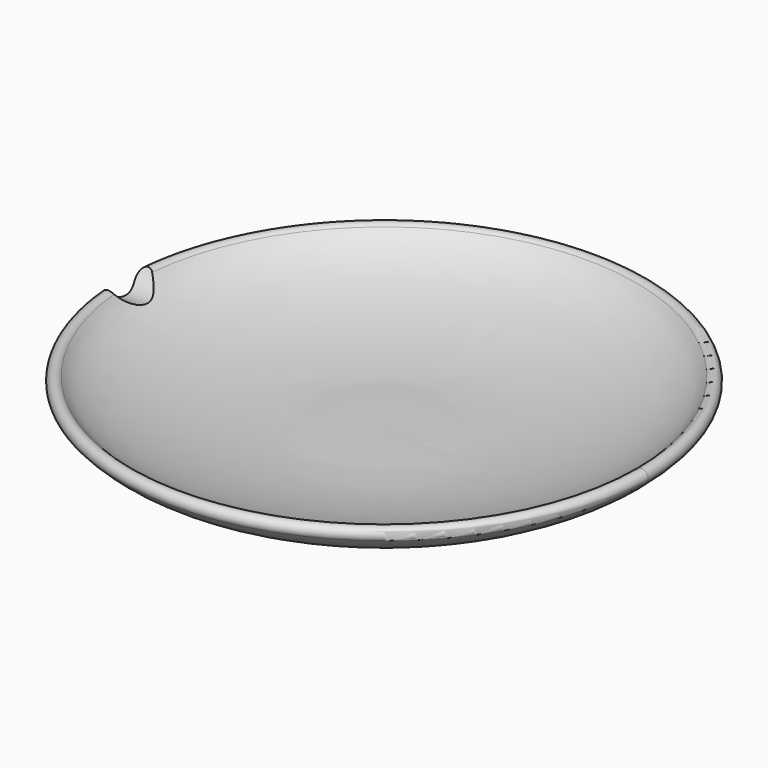
from build123d import *

# Parameters (mm, degrees)
F2_R     = 90.375022763
F3_DEPTH = 2.54
F4_R     = 6.7588472291
F5_DEPTH = 68.326


# Not quite as in the source:
# - the dataset's text gives a spline's control points without its knots; the knots are read off the source's solid


with BuildPart() as f1:
    # F0 (on Front) → F1 (revolve)
    with BuildSketch(Plane.XZ):
        with BuildLine():
            Line((0, 3.175), (0, 0))
            add(Edge.make_bspline(
                [(0, 0), (2.1279627901, 0), (5.8288864996, 0.0050250413), (10.008239819, 0.0167268793), (12.5887522081, 0.0208927398), (14.253408796, 0.0154280645), (15.3378595888, 0.005935087), (16.292128562, -0.0111780463), (17.2331713238, -0.0306431051), (18.2347085448, -0.041814641), (19.358501315, -0.0340795323), (20.6679615044, 0.002626221), (22.2203065643, 0.0764040524), (23.9881376155, 0.1903674356), (26.6029819041, 0.4010278643), (30.2910360113, 0.783807386), (35.1815241674, 1.465523568), (40.329598221, 2.4021546236), (45.5283873865, 3.6305450463), (50.5526729375, 5.170740641), (55.1960014321, 7.0569143003), (58.5913689589, 8.9735205784), (60.9310558305, 10.8006096923), (61.9533690783, 11.8398711964), (62.4180824862, 12.3988049396)],
                knots=[0, 0, 0, 0, 0.0625, 0.125, 0.1875, 0.21875, 0.25, 0.28125, 0.3125, 0.34375, 0.375, 0.40625, 0.4375, 0.46875, 0.5, 0.5625, 0.625, 0.6875, 0.75, 0.8125, 0.875, 0.9375, 0.96875, 1, 1, 1, 1], degree=3))
            ThreePointArc((62.4180824863, 12.3988049396), (62.212308173, 14.6344188222), (59.9766942904, 14.428644509))
            add(Edge.make_bspline(
                [(0, 3.175), (8.8246788449, 3.175), (15.0952757092, 3.2420354498), (20.7728227396, 2.9981599321), (40.7306593531, 4.7042120003), (56.5739250903, 10.3359661101), (59.9766942904, 14.428644509)],
                knots=[0, 0, 0, 0, 0.2594926308, 0.4022821561, 0.6967321573, 1, 1, 1, 1], degree=3))
        make_face()
    revolve(axis=Axis((0, 0, 1.5875), (0, 0, 1)))

    # F2 (on Top) → F3 (cut, symmetric)
    with BuildSketch(Plane.XY):
        Circle(F2_R)
    extrude(amount=F3_DEPTH, both=True, mode=Mode.SUBTRACT)

    # F4 (on Right) → F5 (cut)
    with BuildSketch(Plane.YZ):
        with Locations((0, 18.1135945022)):
            Circle(F4_R)
    extrude(amount=-F5_DEPTH, mode=Mode.SUBTRACT)


solid = f1.part
